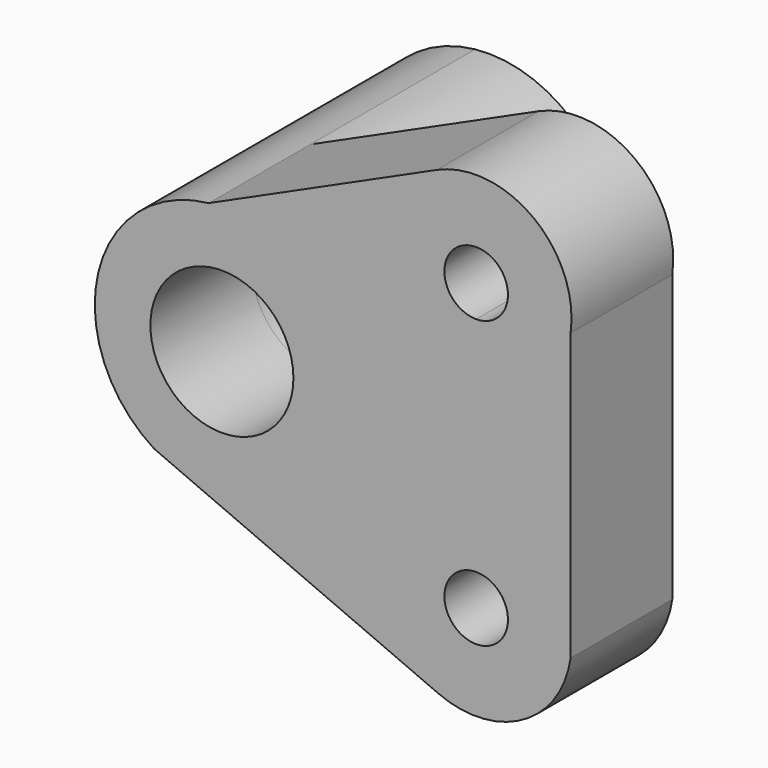
from build123d import *

# Parameters (mm, degrees)
F0_R     = 14.2875
F1_DEPTH = 25.4
F2_DEPTH = 41.148
F3_DEPTH = 40.64
F5_DEPTH = 25.4


with BuildPart() as f1:
    # F0 (on Front) → F1 (new body)
    with BuildSketch(Plane.XZ):
        with BuildLine():
            Line((0, -6.5761469305), (0, 0))
            Line((0, 0), (0, 6.4793750644))
            Line((0, 6.4793750644), (3.6195983623, 6.4793750644))
            ThreePointArc((3.6195983623, 6.4793750644), (-6.5097266562, 20.9027501202), (-23.5870965608, 25.2616961481))
            ThreePointArc((-23.5870965608, 25.2616961481), (-45.6748305827, 5.7751199465), (-34.4999026403, -21.4776896658))
            Line((-34.4999026403, -21.4776896658), (-27.3168603147, -24.5865135025))
            ThreePointArc((-27.3168603147, -24.5865135025), (-8.1528212193, -21.9464362992), (3.5938637092, -6.5761469305))
            Line((3.5938637092, -6.5761469305), (0, -6.5761469305))
        make_face()
        with Locations((-20.9400779136, 0)):
            Circle(F0_R, mode=Mode.SUBTRACT)
        with BuildLine():
            Line((0, 6.4793750644), (0, 0))
            Line((0, 0), (4.4599220864, 0))
            ThreePointArc((4.4599220864, 0), (4.2489651152, 3.2668197527), (3.6195983623, 6.4793750644))
            Line((3.6195983623, 6.4793750644), (0, 6.4793750644))
        make_face()
        with BuildLine():
            Line((4.4599220864, 0), (0, 0))
            Line((0, 0), (0, -6.5761469305))
            Line((0, -6.5761469305), (3.5938637092, -6.5761469305))
            ThreePointArc((3.5938637092, -6.5761469305), (4.2424767346, -3.3164651952), (4.4599220864, 0))
        make_face()
        with BuildLine():
            Line((29.8599220864, 0), (4.4599220864, 0))
            ThreePointArc((4.4599220864, 0), (4.2424767346, -3.3164651952), (3.5938637092, -6.5761469305))
            Line((3.5938637092, -6.5761469305), (48.7220023626, -6.5761469305))
            Line((48.7220023626, -6.5761469305), (48.7220023626, 0))
            Line((48.7220023626, 0), (29.8599220864, 0))
        make_face()
        with BuildLine():
            ThreePointArc((3.6195983623, 6.4793750644), (4.2489651152, 3.2668197527), (4.4599220864, 0))
            Line((4.4599220864, 0), (29.8599220864, 0))
            Line((29.8599220864, 0), (48.7220023626, 0))
            Line((48.7220023626, 0), (48.7220023626, 6.4793750644))
            Line((48.7220023626, 6.4793750644), (3.6195983623, 6.4793750644))
        make_face()
        with BuildLine():
            Line((48.7220023626, -6.5761469305), (3.5938637092, -6.5761469305))
            ThreePointArc((3.5938637092, -6.5761469305), (-8.1528212193, -21.9464362992), (-27.3168603147, -24.5865135025))
            Line((-27.3168603147, -24.5865135025), (22.2933448748, -46.0578318444))
            ThreePointArc((22.2933448748, -46.0578318444), (39.1743355589, -45.1925871192), (48.7220023626, -31.2441623508))
            Line((48.7220023626, -31.2441623508), (48.7220023626, -25.9058376492))
            Line((48.7220023626, -25.9058376492), (48.7220023626, -6.5761469305))
        make_face()
        with BuildLine():
            ThreePointArc((29.8599220864, -22.225), (34.350050147, -24.0848719395), (36.2099220864, -28.575))
            ThreePointArc((36.2099220864, -28.575), (25.3697940259, -33.0651280605), (29.8599220864, -22.225))
        make_face(mode=Mode.SUBTRACT)
        with BuildLine():
            ThreePointArc((-23.5870965608, 25.2616961481), (-6.5097266562, 20.9027501202), (3.6195983623, 6.4793750644))
            Line((3.6195983623, 6.4793750644), (48.7220023626, 6.4793750644))
            Line((48.7220023626, 6.4793750644), (48.7220023626, 25.9058376492))
            ThreePointArc((48.7220023626, 25.9058376492), (41.2803657765, 43.8221625532), (21.9943834178, 45.9253833229))
            Line((21.9943834178, 45.9253833229), (-23.5870965608, 25.2616961481))
        make_face()
        with BuildLine():
            ThreePointArc((29.8599220864, 22.225), (25.3697940259, 33.0651280605), (36.2099220864, 28.575))
            ThreePointArc((36.2099220864, 28.575), (34.350050147, 24.0848719395), (29.8599220864, 22.225))
        make_face(mode=Mode.SUBTRACT)
    extrude(amount=F1_DEPTH)

    # F0 (on Front) → F2 (join)
    with BuildSketch(Plane.XZ):
        with BuildLine():
            Line((0, -6.5761469305), (0, 0))
            Line((0, 0), (0, 6.4793750644))
            Line((0, 6.4793750644), (3.6195983623, 6.4793750644))
            ThreePointArc((3.6195983623, 6.4793750644), (-6.5097266562, 20.9027501202), (-23.5870965608, 25.2616961481))
            ThreePointArc((-23.5870965608, 25.2616961481), (-45.6748305827, 5.7751199465), (-34.4999026403, -21.4776896658))
            Line((-34.4999026403, -21.4776896658), (-27.3168603147, -24.5865135025))
            ThreePointArc((-27.3168603147, -24.5865135025), (-8.1528212193, -21.9464362992), (3.5938637092, -6.5761469305))
            Line((3.5938637092, -6.5761469305), (0, -6.5761469305))
        make_face()
        with Locations((-20.9400779136, 0)):
            Circle(F0_R, mode=Mode.SUBTRACT)
    extrude(amount=-F2_DEPTH)


with BuildPart() as f3:
    # F0 (on Front) → F3 (new body)
    with BuildSketch(Plane.XZ):
        with BuildLine():
            Line((29.8599220864, 0), (4.4599220864, 0))
            ThreePointArc((4.4599220864, 0), (4.2424767346, -3.3164651952), (3.5938637092, -6.5761469305))
            Line((3.5938637092, -6.5761469305), (48.7220023626, -6.5761469305))
            Line((48.7220023626, -6.5761469305), (48.7220023626, 0))
            Line((48.7220023626, 0), (29.8599220864, 0))
        make_face()
        with BuildLine():
            ThreePointArc((3.6195983623, 6.4793750644), (4.2489651152, 3.2668197527), (4.4599220864, 0))
            Line((4.4599220864, 0), (29.8599220864, 0))
            Line((29.8599220864, 0), (48.7220023626, 0))
            Line((48.7220023626, 0), (48.7220023626, 6.4793750644))
            Line((48.7220023626, 6.4793750644), (3.6195983623, 6.4793750644))
        make_face()
    extrude(amount=-F3_DEPTH)

    # F4 (on face) → F5 (cut)
    with BuildSketch(Plane.XY.offset(6.4793750644)):
        Polygon((48.7220023626, 40.64), (3.6195983623, 40.64), (48.7220023626, 0), align=None)
    extrude(amount=-F5_DEPTH, mode=Mode.SUBTRACT)


solid = Compound([f1.part, f3.part])
